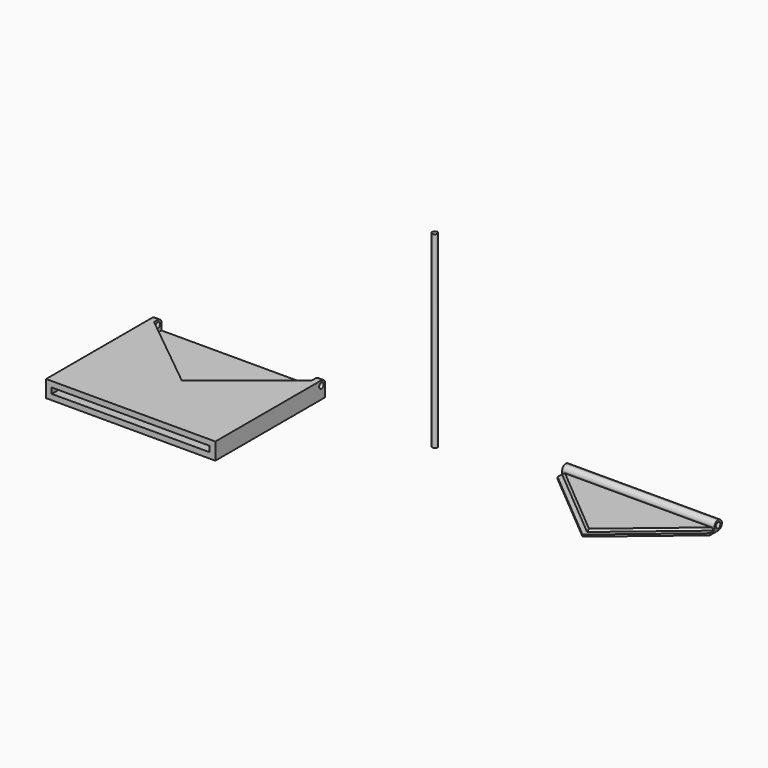
from build123d import *

# Parameters (mm, degrees)
F0_W      = 2286
F0_H      = 1727.2
F1_DEPTH  = 76.2
F2_W      = 76.2
F2_H      = 1727.2
F3_DEPTH  = 76.2
F5_START  = 76.2
F4_W      = 76.2
F4_H      = 1727.2
F5_DEPTH  = 76.2
F6_W      = 2133.6
F6_H      = 76.2
F7_DEPTH  = 127
F9_R      = 38.1
F10_DEPTH = 2291.08
F12_DEPTH = 50.8
F13_DEPTH = 25.4
F11_W     = 2057.4
F11_H     = 127
F14_DEPTH = 127
F15_R     = 38.1
F16_DEPTH = 2276.856
F17_R     = 63.49999
F18_SIZE  = 25.39999
F19_SIZE  = 25.39999
F20_R     = 63.5
F21_R     = 35.56
F22_DEPTH = 2540


# Not quite as in the source:
# - a fillet or chamfer is up to 0.001 mm smaller than in the source, because OpenCascade refuses the exact size


with BuildPart() as f1:
    # F0 (on Top) → F1 (new body)
    with BuildSketch(Plane.XY):
        Rectangle(F0_W, F0_H)
    extrude(amount=F1_DEPTH)

    # F2 (on face) → F3 (join)
    with BuildSketch(Plane.XY.offset(76.2)):
        with Locations((-1104.9, 0)):
            Rectangle(F2_W, F2_H)
        with Locations((1104.9, 0)):
            Rectangle(F2_W, F2_H)
    extrude(amount=F3_DEPTH)

    # F4 (on face) → F5 (join)
    with BuildSketch(Plane.XY.offset(76.2).offset(F5_START)):
        with Locations((-1104.9, 0)):
            Rectangle(F4_W, F4_H)
        with Locations((1104.9, 0)):
            Rectangle(F4_W, F4_H)
        Polygon((-1066.8, 863.6), (-1066.8, -863.6), (1066.8, -863.6), (1066.8, 863.6), (0, 0), align=None)
    extrude(amount=F5_DEPTH)

    # F6 (on face) → F7 (join)
    with BuildSketch(Plane(origin=(0, 863.6, 0), x_dir=(-1, 0, 0), z_dir=(0, 1, 0))):
        Polygon((-1143, 228.6), (-1143, 0), (-1066.8, 0), (-1066.8, 76.2), (-1066.8, 152.4), (-1066.8, 228.6), align=None)
        Polygon((1066.8, 76.2), (1066.8, 0), (1143, 0), (1143, 228.6), (1066.8, 228.6), (1066.8, 152.4), align=None)
        with Locations((0, 38.1)):
            Rectangle(F6_W, F6_H)
    extrude(amount=F7_DEPTH)

    # F9 (on face) → F10 (cut)
    with BuildSketch(Plane.YZ.offset(1143)):
        with Locations((927.1, 165.1)):
            Circle(F9_R)
    extrude(amount=-F10_DEPTH, mode=Mode.SUBTRACT)

    # F20
    f20_edges = [f1.edges().sort_by_distance(p)[0] for p in [
        (-1104.9, 990.6, 228.6),
        (1104.9, 990.6, 228.6),
    ]]
    fillet(f20_edges, radius=F20_R)


with BuildPart() as f12:
    # F11 (on face) → F12 (new body)
    with BuildSketch(Plane.XY.offset(76.2)):
        Polygon((6371.3324619645, 1025.3038924217), (4313.9324619645, 1025.3038924217), (5342.6324619645, 161.7038924217), align=None)
    extrude(amount=F12_DEPTH)

    # F11 (on face) → F13 (join)
    with BuildSketch(Plane.XY.offset(76.2)):
        Polygon((5342.6324619645, 161.7038924217), (4313.9324619645, 1025.3038924217), (4313.9324619645, 949.1038924217), (5251.8648149057, 161.7038924217), align=None)
        Polygon((6371.3324619645, 949.1038924217), (6371.3324619645, 1025.3038924217), (5342.6324619645, 161.7038924217), (5433.4001090233, 161.7038924217), align=None)
        Polygon((5433.4001090233, 161.7038924217), (5342.6324619645, 161.7038924217), (5342.6324619645, 85.5038924217), align=None)
        Polygon((5342.6324619645, 85.5038924217), (5342.6324619645, 161.7038924217), (5251.8648149057, 161.7038924217), align=None)
    extrude(amount=F13_DEPTH)

    # F11 (on face) → F14 (join)
    with BuildSketch(Plane.XY.offset(76.2)):
        with Locations((5342.6324619645, 1088.8038924217)):
            Rectangle(F11_W, F11_H)
    extrude(amount=F14_DEPTH)

    # F15 (on face) → F16 (cut)
    with BuildSketch(Plane.YZ.offset(6371.3324619645)):
        with Locations((1088.8038924217, 139.7)):
            Circle(F15_R)
    extrude(amount=-F16_DEPTH, mode=Mode.SUBTRACT)

    # F17 (radius 63.5 in the source; OpenCascade refuses exactly that, so slightly less here)
    f17_edges = [f12.edges().sort_by_distance(p)[0] for p in [
        (5342.632462, 1152.303892, 203.2),
        (5342.632462, 1025.303892, 203.2),
        (5342.632462, 1152.303892, 76.2),
    ]]
    fillet(f17_edges, radius=F17_R)

    # F18 (size 25.4 in the source; OpenCascade refuses exactly that, so slightly less here)
    f18_edges = [f12.edges().sort_by_distance(p)[0] for p in [
        (4828.282462, 593.503892, 127),
    ]]
    chamfer(f18_edges, length=F18_SIZE)

    # F19 (size 25.4 in the source; OpenCascade refuses exactly that, so slightly less here)
    f19_edges = [f12.edges().sort_by_distance(p)[0] for p in [
        (5866.858497, 601.794885, 127),
    ]]
    chamfer(f19_edges, length=F19_SIZE)


with BuildPart() as f22:
    # F21 (on face) → F22 (new body)
    with BuildSketch(Plane.XY.offset(76.2)):
        with Locations((2838.5834693909, 722.6612567902)):
            Circle(F21_R)
    extrude(amount=F22_DEPTH)


solid = Compound([f1.part, f12.part, f22.part])
